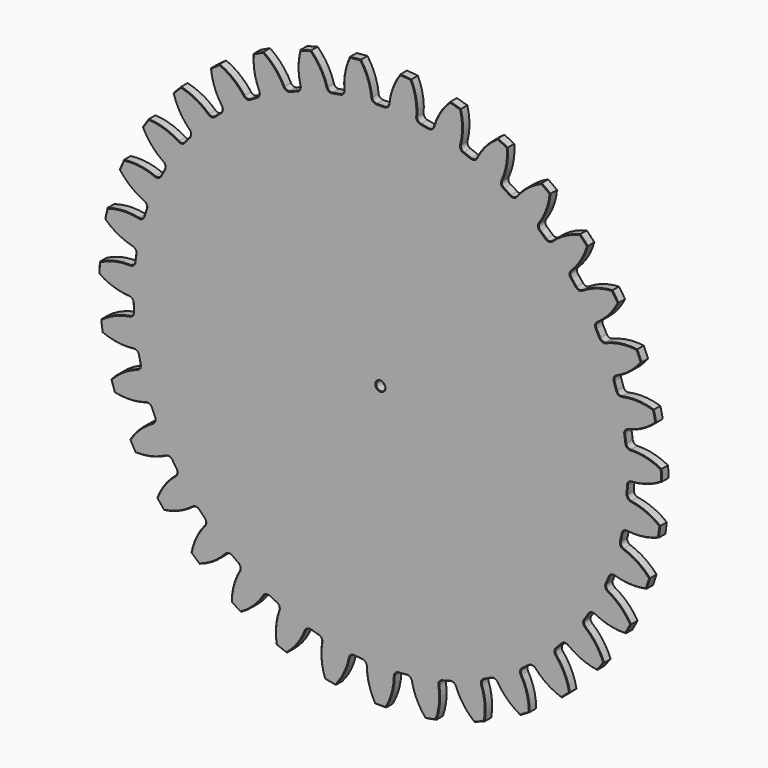
from build123d import *

# Parameters (mm, degrees)
F2_R            = 92.5
F2_R_2          = 87.5
F2_R_3          = 81.25
F3_DEPTH        = 1.5
F4_R            = 1.5
F5_DEPTH        = 1.501
F5_DEPTH_BACK   = 1.501
F7_DEPTH        = 1.501
F7_DEPTH_BACK   = 1.501
F7_COPIES_COUNT = 35
F8_R            = 1.5
F9_SIZE         = 0.18


# Not quite as in the source:
# - a pattern or mirror of a feature is missing from the dataset's text; its kind, count and spacing are read off the source's solid


with BuildPart() as f3:
    # F2 (on Front) → F3 (new body, symmetric)
    with BuildSketch(Plane.XZ):
        Circle(F2_R)
        Circle(F2_R_2, mode=Mode.SUBTRACT)
        Circle(F2_R_2)
        Circle(F2_R_3, mode=Mode.SUBTRACT)
        Circle(F2_R_3)
    extrude(amount=F3_DEPTH, both=True)

    # F4 (on Front) → F5 (cut, two sides)
    with BuildSketch(Plane.XZ) as f5_sk:
        Circle(F4_R)
    extrude(amount=-F5_DEPTH, mode=Mode.SUBTRACT)
    extrude(f5_sk.sketch, amount=F5_DEPTH_BACK, mode=Mode.SUBTRACT)

    # F6 (on Front) → F7 (cut, two sides)
    with BuildSketch(Plane.XZ) as f7_sk:
        with BuildLine():
            ThreePointArc((-7.2191244755, 93.2208895141), (-3.9879045768, 87.5805267005), (-2.7234925528, 81.2043415607))
            ThreePointArc((-2.7234925528, 81.2043415607), (0, 81.25), (2.7234925528, 81.2043415607))
            ThreePointArc((2.7234925528, 81.2043415607), (3.9879045768, 87.5805267005), (7.2191244755, 93.2208895141))
            ThreePointArc((7.2191244755, 93.2208895141), (0, 93.5), (-7.2191244755, 93.2208895141))
        make_face()
    f7 = extrude(amount=-F7_DEPTH, mode=Mode.SUBTRACT) + extrude(f7_sk.sketch, amount=F7_DEPTH_BACK, mode=Mode.SUBTRACT)

    # F7_copies: F7 ×35 about axis
    f7_copies_axis = Axis((0, 0, 0), (0, 1, 0))
    for i in range(1, F7_COPIES_COUNT):
        add(f7.rotate(f7_copies_axis, i * 360 / F7_COPIES_COUNT), mode=Mode.SUBTRACT)

    # F8
    f8_edges = [f3.edges().sort_by_distance(p)[0] for p in [
        (-2.723493, 0, 81.204342),
        (2.723493, 0, 81.204342),
        (17.17932, 0, 79.413056),
        (25.983333, 0, 76.983303),
        (11.81987, 0, 80.385653),
        (80.10384, 0, 13.599168),
        (80.835006, 0, 8.20148),
        (81.244763, 0, -0.922469),
        (81.000385, 0, -6.363969),
        (79.774413, 0, -15.414457),
        (78.562345, 0, -20.724875),
        (75.740048, 0, -29.411012),
        (73.599247, 0, -34.419666),
        (69.271335, 0, -42.462273),
        (66.270608, 0, -47.008181),
        (60.576185, 0, -54.148761),
        (56.811977, 0, -58.085814),
        (49.934066, 0, -64.094864),
        (45.527363, 0, -67.296521),
        (37.687025, 0, -71.980905),
        (32.779461, 0, -74.344263),
        (24.228693, 0, -77.55342),
        (18.978001, 0, -79.002519),
        (9.99163, 0, -80.633305),
        (4.566572, 0, -81.121569),
        (-4.566572, 0, -81.121569),
        (-9.99163, 0, -80.633305),
        (-18.978001, 0, -79.002519),
        (-24.228693, 0, -77.55342),
        (-32.779461, 0, -74.344263),
        (-37.687025, 0, -71.980905),
        (-45.527363, 0, -67.296521),
        (-49.934066, 0, -64.094864),
        (-56.811977, 0, -58.085814),
        (-60.576185, 0, -54.148761),
        (-66.270608, 0, -47.008181),
        (-69.271335, 0, -42.462273),
        (-73.599247, 0, -34.419666),
        (-75.740048, 0, -29.411012),
        (-78.562345, 0, -20.724875),
        (-79.774413, 0, -15.414457),
        (-81.000385, 0, -6.363969),
        (-81.244763, 0, -0.922469),
        (-80.835006, 0, 8.20148),
        (-80.10384, 0, 13.599168),
        (-78.071524, 0, 22.503326),
        (-76.388313, 0, 27.683717),
        (-72.798758, 0, 36.081897),
        (-70.217603, 0, 40.878488),
        (-65.186181, 0, 48.500767),
        (-61.790041, 0, 52.759391),
        (-55.478466, 0, 59.360781),
        (-51.376496, 0, 62.944564),
        (-43.987627, 0, 68.312892),
        (-39.311669, 0, 71.106646),
        (-31.08299, 0, 75.069369),
        (-25.983333, 0, 76.983303),
        (-17.17932, 0, 79.413056),
        (-11.81987, 0, 80.385653),
        (31.08299, 0, 75.069369),
        (39.311669, 0, 71.106646),
        (43.987627, 0, 68.312892),
        (51.376496, 0, 62.944564),
        (55.478466, 0, 59.360781),
        (61.790041, 0, 52.759391),
        (65.186181, 0, 48.500767),
        (70.217603, 0, 40.878488),
        (72.798758, 0, 36.081897),
        (76.388313, 0, 27.683717),
        (78.071524, 0, 22.503326),
    ]]
    fillet(f8_edges, radius=F8_R)

    # F9
    f9_edges = [f3.edges().sort_by_distance(p)[0] for p in [
        (27.039851, -1.5, 83.492355),
        (26.505047, -1.5, 77.229157),
        (24.608408, -1.5, 89.166565),
        (28.549204, -1.5, 76.069083),
        (19.610841, -1.5, 85.542631),
        (30.851859, -1.5, 75.597771),
        (16.857553, -1.5, 79.891696),
        (34.569913, -1.5, 80.666275),
        (14.507748, -1.5, 79.944279),
        (40.134246, -1.5, 83.33962),
        (12.289301, -1.5, 80.720711),
        (41.513445, -1.5, 77.322447),
        (11.697174, -1.5, 86.97875),
        (39.868898, -1.5, 71.255394),
        (8.291636, -1.5, 92.127622),
        (41.673066, -1.5, 69.748964),
        (4.02146, -1.5, 87.669577),
        (43.85456, -1.5, 68.874072),
        (2.321432, -1.5, 81.617836),
        (48.41788, -1.5, 73.197238),
        (0, -1.5, 81.25),
        (54.370136, -1.5, 74.834072),
        (-2.321432, -1.5, 81.617836),
        (54.652763, -1.5, 68.667331),
        (-4.02146, -1.5, 87.669577),
        (51.95133, -1.5, 62.991424),
        (-8.291636, -1.5, 92.127622),
        (53.457521, -1.5, 61.187057),
        (-11.697174, -1.5, 86.97875),
        (55.447739, -1.5, 59.936703),
        (-12.289301, -1.5, 80.720711),
        (60.709657, -1.5, 63.375582),
        (-14.507748, -1.5, 79.944279),
        (66.858525, -1.5, 63.923295),
        (-16.857553, -1.5, 79.891696),
        (66.035496, -1.5, 57.805191),
        (-19.610841, -1.5, 85.542631),
        (62.364004, -1.5, 52.702857),
        (-24.608408, -1.5, 89.166565),
        (63.523808, -1.5, 50.658546),
        (-27.039851, -1.5, 83.492355),
        (65.258783, -1.5, 49.072919),
        (-26.505047, -1.5, 77.229157),
        (71.050175, -1.5, 51.516983),
        (-28.549204, -1.5, 76.069083),
        (77.198026, -1.5, 50.957971),
        (-30.851859, -1.5, 75.597771),
        (75.295794, -1.5, 45.085145),
        (-34.569913, -1.5, 80.666275),
        (70.772247, -1.5, 40.720378),
        (-40.134246, -1.5, 83.33962),
        (71.548387, -1.5, 38.501829),
        (-41.513445, -1.5, 77.322447),
        (72.972356, -1.5, 36.631892),
        (-39.868898, -1.5, 71.255394),
        (79.107082, -1.5, 38.002585),
        (-41.673066, -1.5, 69.748964),
        (85.056319, -1.5, 36.354815),
        (-43.85456, -1.5, 68.874072),
        (82.136023, -1.5, 30.916025),
        (-48.41788, -1.5, 73.197238),
        (76.905812, -1.5, 27.429112),
        (-54.370136, -1.5, 74.834072),
        (77.273342, -1.5, 25.107631),
        (-54.652763, -1.5, 68.667331),
        (78.340537, -1.5, 23.013485),
        (-51.95133, -1.5, 62.991424),
        (84.621422, -1.5, 23.266753),
        (-53.457521, -1.5, 61.187057),
        (90.180832, -1.5, 20.583186),
        (-55.447739, -1.5, 59.936703),
        (86.336333, -1.5, 15.753239),
        (-60.709657, -1.5, 63.375582),
        (80.567561, -1.5, 13.256252),
        (-66.858525, -1.5, 63.923295),
        (80.514668, -1.5, 10.906453),
        (-66.035496, -1.5, 57.805191),
        (81.190788, -1.5, 8.655406),
        (-62.364004, -1.5, 52.702857),
        (87.41596, -1.5, 7.783109),
        (-63.523808, -1.5, 50.658546),
        (92.406859, -1.5, 4.149997),
        (-65.258783, -1.5, 49.072919),
        (87.761722, -1.5, 0.08413),
        (-71.050175, -1.5, 51.516983),
        (81.639803, -1.5, -1.342675),
        (-77.198026, -1.5, 50.957971),
        (81.168187, -1.5, -3.645267),
        (-75.295794, -1.5, 45.085145),
        (81.431501, -1.5, -5.980865),
        (-70.772247, -1.5, 40.720378),
        (87.400877, -1.5, -7.950692),
        (-71.548387, -1.5, 38.501829),
        (91.662853, -1.5, -12.416577),
        (-72.972356, -1.5, 36.631892),
        (86.366377, -1.5, -15.587682),
        (-79.107082, -1.5, 38.002585),
        (80.088074, -1.5, -15.898448),
        (-85.056319, -1.5, 36.354815),
        (79.212893, -1.5, -18.079826),
        (-82.136023, -1.5, 30.916025),
        (79.054939, -1.5, -20.424906),
        (-76.905812, -1.5, 27.429112),
        (84.576658, -1.5, -23.42895),
        (-77.273342, -1.5, 25.107631),
        (87.972728, -1.5, -28.584072),
        (-78.340537, -1.5, 23.013485),
        (82.195145, -1.5, -30.758494),
        (-84.621422, -1.5, 23.266753),
        (75.962248, -1.5, -29.943231),
        (-90.180832, -1.5, 20.583186),
        (74.711632, -1.5, -31.933284),
        (-86.336333, -1.5, 15.753239),
        (74.137486, -1.5, -34.212474),
        (-80.567561, -1.5, 13.256252),
        (79.034076, -1.5, -38.154183),
        (-80.514668, -1.5, 10.906453),
        (81.455087, -1.5, -43.832851),
        (-81.190788, -1.5, 8.655406),
        (75.382094, -1.5, -44.940702),
        (-87.41596, -1.5, 7.783109),
        (69.394933, -1.5, -43.025614),
        (-92.406859, -1.5, 4.149997),
        (67.809077, -1.5, -44.76038),
        (-87.761722, -1.5, 0.08413),
        (66.837193, -1.5, -46.900425),
        (-81.639803, -1.5, -1.342675),
        (70.951274, -1.5, -51.653108),
        (-81.168187, -1.5, -3.645267),
        (72.319412, -1.5, -57.672807),
        (-81.431501, -1.5, -5.980865),
        (66.146201, -1.5, -57.678479),
        (-87.400877, -1.5, -7.950692),
        (60.597208, -1.5, -54.725118),
        (-91.662853, -1.5, -12.416577),
        (58.727083, -1.5, -56.14884),
        (-86.366377, -1.5, -15.587682),
        (57.388697, -1.5, -58.080957),
        (-80.088074, -1.5, -15.898448),
        (60.588039, -1.5, -63.491861),
        (-79.212893, -1.5, -18.079826),
        (60.859332, -1.5, -69.659111),
        (-79.054939, -1.5, -20.424906),
        (54.784314, -1.5, -68.562422),
        (-84.576658, -1.5, -23.42895),
        (49.851838, -1.5, -64.665712),
        (-87.972728, -1.5, -28.584072),
        (47.757552, -1.5, -65.732631),
        (-82.195145, -1.5, -30.758494),
        (46.095682, -1.5, -67.39472),
        (-75.962248, -1.5, -29.943231),
        (48.277455, -1.5, -73.289933),
        (-74.711632, -1.5, -31.933284),
        (47.443183, -1.5, -79.406513),
        (-74.137486, -1.5, -34.212474),
        (41.661614, -1.5, -77.242713),
        (-79.034076, -1.5, -38.154183),
        (37.50419, -1.5, -72.527897),
        (-81.455087, -1.5, -43.832851),
        (35.253054, -1.5, -73.203721),
        (-75.382094, -1.5, -44.940702),
        (33.321113, -1.5, -74.542361),
        (-69.394933, -1.5, -43.025614),
        (34.415193, -1.5, -80.732406),
        (-67.809077, -1.5, -44.76038),
        (32.502171, -1.5, -86.601726),
        (-66.837193, -1.5, -46.900425),
        (27.199876, -1.5, -83.440359),
        (-70.951274, -1.5, -51.653108),
        (23.951126, -1.5, -78.058976),
        (-72.319412, -1.5, -57.672807),
        (21.615494, -1.5, -78.321982),
        (-66.146201, -1.5, -57.678479),
        (19.475577, -1.5, -79.294149),
        (-60.597208, -1.5, -54.725118),
        (19.446799, -1.5, -85.580073),
        (-58.727083, -1.5, -56.14884),
        (16.516513, -1.5, -91.013487),
        (-57.388697, -1.5, -58.080957),
        (11.863911, -1.5, -86.956164),
        (-60.588039, -1.5, -63.491861),
        (9.628253, -1.5, -81.081175),
        (-60.859332, -1.5, -69.659111),
        (7.283194, -1.5, -80.922911),
        (-54.784314, -1.5, -68.562422),
        (5.004079, -1.5, -81.497358),
        (-49.851838, -1.5, -64.665712),
        (3.853369, -1.5, -87.677126),
        (-47.757552, -1.5, -65.732631),
        (0, -1.5, -92.5),
        (-46.095682, -1.5, -67.39472),
        (-3.853369, -1.5, -87.677126),
        (-48.277455, -1.5, -73.289933),
        (-5.004079, -1.5, -81.497358),
        (-47.443183, -1.5, -79.406513),
        (-7.283194, -1.5, -80.922911),
        (-41.661614, -1.5, -77.242713),
        (-9.628253, -1.5, -81.081175),
        (-37.50419, -1.5, -72.527897),
        (-11.863911, -1.5, -86.956164),
        (-35.253054, -1.5, -73.203721),
        (-16.516513, -1.5, -91.013487),
        (-33.321113, -1.5, -74.542361),
        (-19.446799, -1.5, -85.580073),
        (-34.415193, -1.5, -80.732406),
        (-19.475577, -1.5, -79.294149),
        (-32.502171, -1.5, -86.601726),
        (-21.615494, -1.5, -78.321982),
        (-27.199876, -1.5, -83.440359),
        (-23.951126, -1.5, -78.058976),
        (-1.5, -1.5, 0),
        (80.514668, 1.5, 10.906453),
        (81.190788, 1.5, 8.655406),
        (80.567561, 1.5, 13.256252),
        (87.41596, 1.5, 7.783109),
        (86.336333, 1.5, 15.753239),
        (92.406859, 1.5, 4.149997),
        (90.180832, 1.5, 20.583186),
        (87.761722, 1.5, 0.08413),
        (84.621422, 1.5, 23.266753),
        (81.639803, 1.5, -1.342675),
        (78.340537, 1.5, 23.013485),
        (81.168187, 1.5, -3.645267),
        (77.273342, 1.5, 25.107631),
        (81.431501, 1.5, -5.980865),
        (76.905812, 1.5, 27.429112),
        (87.400877, 1.5, -7.950692),
        (82.136023, 1.5, 30.916025),
        (91.662853, 1.5, -12.416577),
        (85.056319, 1.5, 36.354815),
        (86.366377, 1.5, -15.587682),
        (79.107082, 1.5, 38.002585),
        (80.088074, 1.5, -15.898448),
        (72.972356, 1.5, 36.631892),
        (79.212893, 1.5, -18.079826),
        (71.548387, 1.5, 38.501829),
        (79.054939, 1.5, -20.424906),
        (70.772247, 1.5, 40.720378),
        (84.576658, 1.5, -23.42895),
        (75.295794, 1.5, 45.085145),
        (87.972728, 1.5, -28.584072),
        (77.198026, 1.5, 50.957971),
        (82.195145, 1.5, -30.758494),
        (71.050175, 1.5, 51.516983),
        (75.962248, 1.5, -29.943231),
        (65.258783, 1.5, 49.072919),
        (74.711632, 1.5, -31.933284),
        (63.523808, 1.5, 50.658546),
        (74.137486, 1.5, -34.212474),
        (62.364004, 1.5, 52.702857),
        (79.034076, 1.5, -38.154183),
        (66.035496, 1.5, 57.805191),
        (81.455087, 1.5, -43.832851),
        (66.858525, 1.5, 63.923295),
        (75.382094, 1.5, -44.940702),
        (60.709657, 1.5, 63.375582),
        (69.394933, 1.5, -43.025614),
        (55.447739, 1.5, 59.936703),
        (67.809077, 1.5, -44.76038),
        (53.457521, 1.5, 61.187057),
        (66.837193, 1.5, -46.900425),
        (51.95133, 1.5, 62.991424),
        (70.951274, 1.5, -51.653108),
        (54.652763, 1.5, 68.667331),
        (72.319412, 1.5, -57.672807),
        (54.370136, 1.5, 74.834072),
        (66.146201, 1.5, -57.678479),
        (48.41788, 1.5, 73.197238),
        (60.597208, 1.5, -54.725118),
        (43.85456, 1.5, 68.874072),
        (58.727083, 1.5, -56.14884),
        (41.673066, 1.5, 69.748964),
        (57.388697, 1.5, -58.080957),
        (39.868898, 1.5, 71.255394),
        (60.588039, 1.5, -63.491861),
        (41.513445, 1.5, 77.322447),
        (60.859332, 1.5, -69.659111),
        (40.134246, 1.5, 83.33962),
        (54.784314, 1.5, -68.562422),
        (34.569913, 1.5, 80.666275),
        (49.851838, 1.5, -64.665712),
        (30.851859, 1.5, 75.597771),
        (47.757552, 1.5, -65.732631),
        (28.549204, 1.5, 76.069083),
        (46.095682, 1.5, -67.39472),
        (26.505047, 1.5, 77.229157),
        (48.277455, 1.5, -73.289933),
        (27.039851, 1.5, 83.492355),
        (47.443183, 1.5, -79.406513),
        (24.608408, 1.5, 89.166565),
        (41.661614, 1.5, -77.242713),
        (19.610841, 1.5, 85.542631),
        (37.50419, 1.5, -72.527897),
        (16.857553, 1.5, 79.891696),
        (35.253054, 1.5, -73.203721),
        (14.507748, 1.5, 79.944279),
        (33.321113, 1.5, -74.542361),
        (12.289301, 1.5, 80.720711),
        (34.415193, 1.5, -80.732406),
        (11.697174, 1.5, 86.97875),
        (32.502171, 1.5, -86.601726),
        (8.291636, 1.5, 92.127622),
        (27.199876, 1.5, -83.440359),
        (4.02146, 1.5, 87.669577),
        (23.951126, 1.5, -78.058976),
        (2.321432, 1.5, 81.617836),
        (21.615494, 1.5, -78.321982),
        (0, 1.5, 81.25),
        (19.475577, 1.5, -79.294149),
        (-2.321432, 1.5, 81.617836),
        (19.446799, 1.5, -85.580073),
        (-4.02146, 1.5, 87.669577),
        (16.516513, 1.5, -91.013487),
        (-8.291636, 1.5, 92.127622),
        (11.863911, 1.5, -86.956164),
        (-11.697174, 1.5, 86.97875),
        (9.628253, 1.5, -81.081175),
        (-12.289301, 1.5, 80.720711),
        (7.283194, 1.5, -80.922911),
        (-14.507748, 1.5, 79.944279),
        (5.004079, 1.5, -81.497358),
        (-16.857553, 1.5, 79.891696),
        (3.853369, 1.5, -87.677126),
        (-19.610841, 1.5, 85.542631),
        (0, 1.5, -92.5),
        (-24.608408, 1.5, 89.166565),
        (-3.853369, 1.5, -87.677126),
        (-27.039851, 1.5, 83.492355),
        (-5.004079, 1.5, -81.497358),
        (-26.505047, 1.5, 77.229157),
        (-7.283194, 1.5, -80.922911),
        (-28.549204, 1.5, 76.069083),
        (-9.628253, 1.5, -81.081175),
        (-30.851859, 1.5, 75.597771),
        (-11.863911, 1.5, -86.956164),
        (-34.569913, 1.5, 80.666275),
        (-16.516513, 1.5, -91.013487),
        (-40.134246, 1.5, 83.33962),
        (-19.446799, 1.5, -85.580073),
        (-41.513445, 1.5, 77.322447),
        (-19.475577, 1.5, -79.294149),
        (-39.868898, 1.5, 71.255394),
        (-21.615494, 1.5, -78.321982),
        (-41.673066, 1.5, 69.748964),
        (-23.951126, 1.5, -78.058976),
        (-43.85456, 1.5, 68.874072),
        (-27.199876, 1.5, -83.440359),
        (-48.41788, 1.5, 73.197238),
        (-32.502171, 1.5, -86.601726),
        (-54.370136, 1.5, 74.834072),
        (-34.415193, 1.5, -80.732406),
        (-54.652763, 1.5, 68.667331),
        (-33.321113, 1.5, -74.542361),
        (-51.95133, 1.5, 62.991424),
        (-35.253054, 1.5, -73.203721),
        (-53.457521, 1.5, 61.187057),
        (-37.50419, 1.5, -72.527897),
        (-55.447739, 1.5, 59.936703),
        (-41.661614, 1.5, -77.242713),
        (-60.709657, 1.5, 63.375582),
        (-47.443183, 1.5, -79.406513),
        (-66.858525, 1.5, 63.923295),
        (-48.277455, 1.5, -73.289933),
        (-66.035496, 1.5, 57.805191),
        (-46.095682, 1.5, -67.39472),
        (-62.364004, 1.5, 52.702857),
        (-47.757552, 1.5, -65.732631),
        (-63.523808, 1.5, 50.658546),
        (-49.851838, 1.5, -64.665712),
        (-65.258783, 1.5, 49.072919),
        (-54.784314, 1.5, -68.562422),
        (-71.050175, 1.5, 51.516983),
        (-60.859332, 1.5, -69.659111),
        (-77.198026, 1.5, 50.957971),
        (-60.588039, 1.5, -63.491861),
        (-75.295794, 1.5, 45.085145),
        (-57.388697, 1.5, -58.080957),
        (-70.772247, 1.5, 40.720378),
        (-58.727083, 1.5, -56.14884),
        (-71.548387, 1.5, 38.501829),
        (-60.597208, 1.5, -54.725118),
        (-72.972356, 1.5, 36.631892),
        (-66.146201, 1.5, -57.678479),
        (-79.107082, 1.5, 38.002585),
        (-72.319412, 1.5, -57.672807),
        (-85.056319, 1.5, 36.354815),
        (-70.951274, 1.5, -51.653108),
        (-82.136023, 1.5, 30.916025),
        (-66.837193, 1.5, -46.900425),
        (-76.905812, 1.5, 27.429112),
        (-67.809077, 1.5, -44.76038),
        (-77.273342, 1.5, 25.107631),
        (-69.394933, 1.5, -43.025614),
        (-78.340537, 1.5, 23.013485),
        (-75.382094, 1.5, -44.940702),
        (-84.621422, 1.5, 23.266753),
        (-81.455087, 1.5, -43.832851),
        (-90.180832, 1.5, 20.583186),
        (-79.034076, 1.5, -38.154183),
        (-86.336333, 1.5, 15.753239),
        (-74.137486, 1.5, -34.212474),
        (-80.567561, 1.5, 13.256252),
        (-74.711632, 1.5, -31.933284),
        (-80.514668, 1.5, 10.906453),
        (-75.962248, 1.5, -29.943231),
        (-81.190788, 1.5, 8.655406),
        (-82.195145, 1.5, -30.758494),
        (-87.41596, 1.5, 7.783109),
        (-87.972728, 1.5, -28.584072),
        (-92.406859, 1.5, 4.149997),
        (-84.576658, 1.5, -23.42895),
        (-87.761722, 1.5, 0.08413),
        (-79.054939, 1.5, -20.424906),
        (-81.639803, 1.5, -1.342675),
        (-79.212893, 1.5, -18.079826),
        (-81.168187, 1.5, -3.645267),
        (-80.088074, 1.5, -15.898448),
        (-81.431501, 1.5, -5.980865),
        (-86.366377, 1.5, -15.587682),
        (-87.400877, 1.5, -7.950692),
        (-91.662853, 1.5, -12.416577),
        (-1.5, 1.5, 0),
    ]]
    chamfer(f9_edges, length=F9_SIZE)


solid = f3.part
